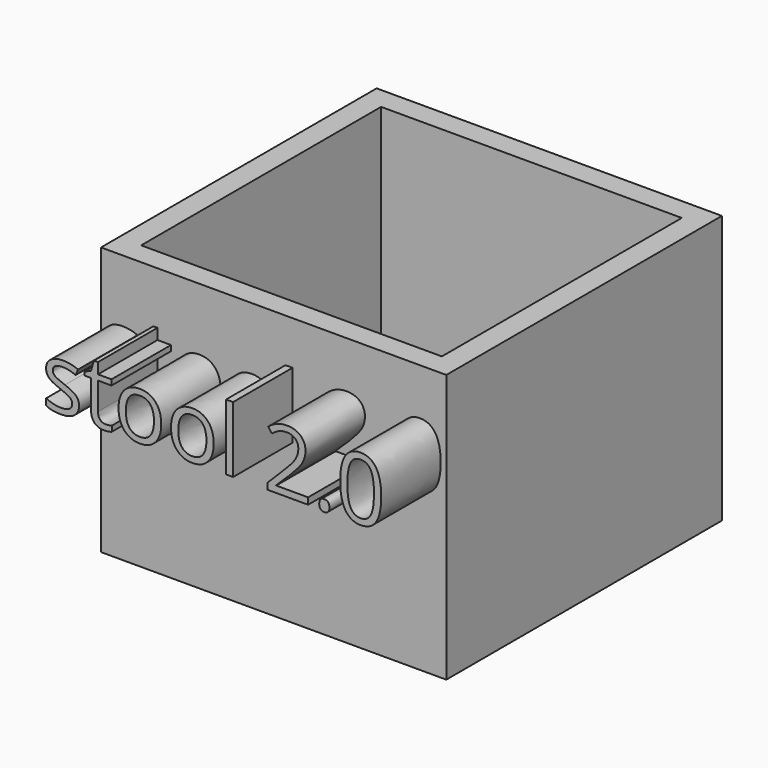
from build123d import *

# Parameters (mm, degrees)
F0_W         = 118.0179789662
F0_H         = 117.7602857351
F1_DEPTH     = 91.694
F3_T         = -7.62
F2_TEXT_SIZE = 29.6853900874
F4_DEPTH     = 25.4


# Not quite as in the source:
# - Text() gives the source's letters only with a copy of the font that has no kerning and outlines rounded to 1/6400 em; it was checked with that copy


with BuildPart() as f1:
    # F0 (on Top) → F1 (new body)
    with BuildSketch(Plane.XY):
        with Locations((17.0069597661, -17.7799984813)):
            Rectangle(F0_W, F0_H)
    extrude(amount=F1_DEPTH)

    # F3
    f3_openings = [f1.faces().sort_by_distance(p)[0] for p in [
        (17.00696, -17.779998, 91.694),
    ]]
    offset(amount=F3_T, openings=f3_openings)

    # F2 (on face) → F4 (join)
    with BuildSketch(Plane.XZ.offset(76.6601413488)):
        with Locations((-42.002029717, 54.2104913769)):
            Text('stool 2.0', F2_TEXT_SIZE, font='Open Sans', text_align=(TextAlign.LEFT, TextAlign.BOTTOM))
    extrude(amount=F4_DEPTH)


solid = f1.part
